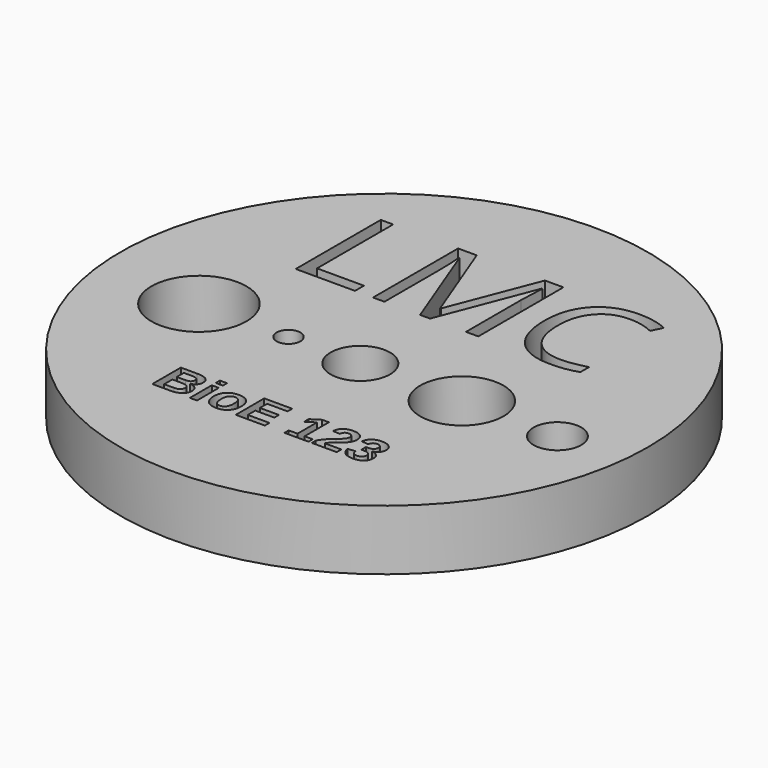
from build123d import *

# Parameters (mm, degrees)
F0_R         = 22.225
F1_DEPTH     = 5.08
F2_R         = 4.0005
F2_R_2       = 1.0033
F2_R_3       = 2.5019
F2_R_4       = 3.5052
F2_R_5       = 2.0066
F3_TEXT_SIZE = 12.5402686082
F4_TEXT_SIZE = 4.3600920921
F5_DEPTH     = 5.081


# Not quite as in the source:
# - Text() gives the source's letters only with a copy of the font that has no kerning and outlines rounded to 1/6400 em; it was checked with that copy


with BuildPart() as f1:
    # F0 (on Top) → F1 (new body)
    with BuildSketch(Plane.XY):
        Circle(F0_R)
    extrude(amount=F1_DEPTH)

    # F2 (on Top) + F3 (on Top) + F4 (on Top) → F5 (cut, through all)
    with BuildSketch(Plane.XY):
        with Locations((-13.589, -2.5019)):
            Circle(F2_R)
        with Locations((-6.0452, -2.5019)):
            Circle(F2_R_2)
        with Locations((0, -2.5019)):
            Circle(F2_R_3)
        with Locations((8.5471, -2.5019)):
            Circle(F2_R_4)
        with Locations((16.5989, -2.5019)):
            Circle(F2_R_5)
    with BuildSketch(Plane.XY):
        with Locations((-12.9483295535, 5.3467)):
            Text('LMC', F3_TEXT_SIZE, font='Open Sans', text_align=(TextAlign.LEFT, TextAlign.BOTTOM))
    with BuildSketch(Plane.XY):
        with Locations((-9.1383295535, -13.3342382126)):
            Text('BioE 123', F4_TEXT_SIZE, font='Arimo', font_style=FontStyle.BOLD, text_align=(TextAlign.LEFT, TextAlign.BOTTOM))
    extrude(amount=F5_DEPTH, mode=Mode.SUBTRACT)


solid = f1.part
